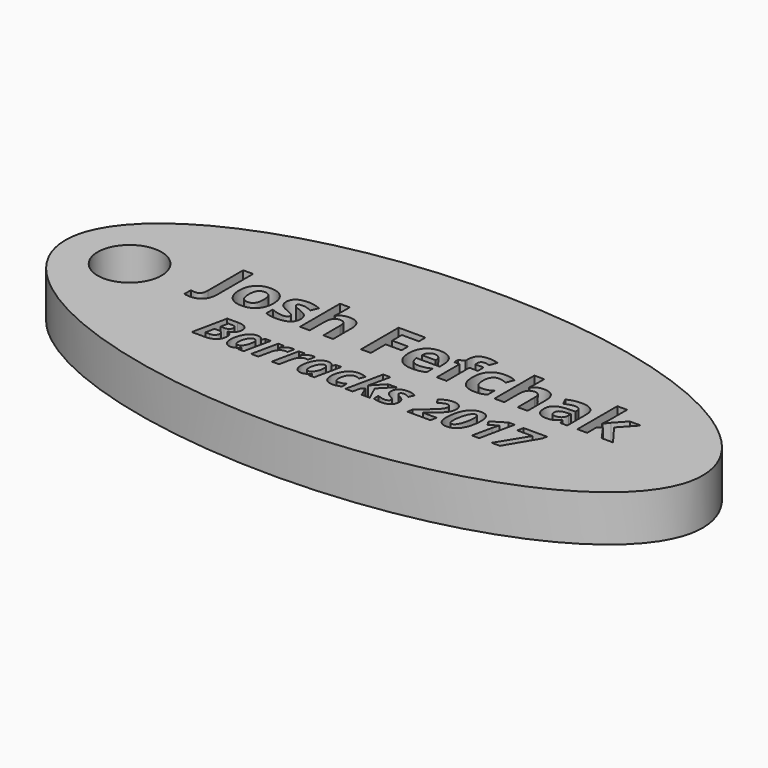
from build123d import *

# Parameters (mm, degrees)
F1_DEPTH     = 4.572
F2_R         = 3.1653305339
F3_DEPTH     = 21.336
F4_TEXT_SIZE = 6.516512445
F5_DEPTH     = 2.032
F6_TEXT_SIZE = 4.8739881565
F7_DEPTH     = 2.032


# Not quite as in the source:
# - Text() gives the source's letters only with a copy of the font that has no kerning and outlines rounded to 1/6400 em; it was checked with that copy


with BuildPart() as f1:
    # F0 (on Top) → F1 (new body)
    with BuildSketch(Plane.XY):
        with BuildLine():
            add(Edge.make_bspline(
                [(-31.5907256366, 0), (-31.5907256366, -24.1462624431), (15.7953628183, -12.0731312216), (63.1814512732, 0), (15.7953628183, 12.0731312216), (-31.5907256366, 24.1462624431), (-31.5907256366, 0)],
                knots=[0, 0, 0, 2.0943951024, 2.0943951024, 4.1887902048, 4.1887902048, 6.2831853072, 6.2831853072, 6.2831853072], degree=2, weights=[1, 0.5, 1, 0.5, 1, 0.5, 1]))
        make_face()
    extrude(amount=F1_DEPTH)

    # F2 (on face) → F3 (cut)
    with BuildSketch(Plane.XY.offset(4.572)):
        with Locations((-25.2246279269, 0)):
            Circle(F2_R)
    extrude(amount=-F3_DEPTH, mode=Mode.SUBTRACT)

    # F4 (on face) → F5 (cut)
    with BuildSketch(Plane.XY.offset(4.572)):
        with Locations((-18.2703510261, 0)):
            Text('Josh Fefchak', F4_TEXT_SIZE, font='Open Sans', font_style=FontStyle.BOLD, text_align=(TextAlign.LEFT, TextAlign.BOTTOM))
    extrude(amount=-F5_DEPTH, mode=Mode.SUBTRACT)

    # F6 (on face) → F7 (cut)
    with BuildSketch(Plane.XY.offset(4.572)):
        with Locations((-14.4491547317, -5.9212218039)):
            Text('Barracks 2017', F6_TEXT_SIZE, font='Open Sans', font_style=FontStyle.BOLDITALIC, text_align=(TextAlign.LEFT, TextAlign.BOTTOM))
    extrude(amount=-F7_DEPTH, mode=Mode.SUBTRACT)


solid = f1.part
